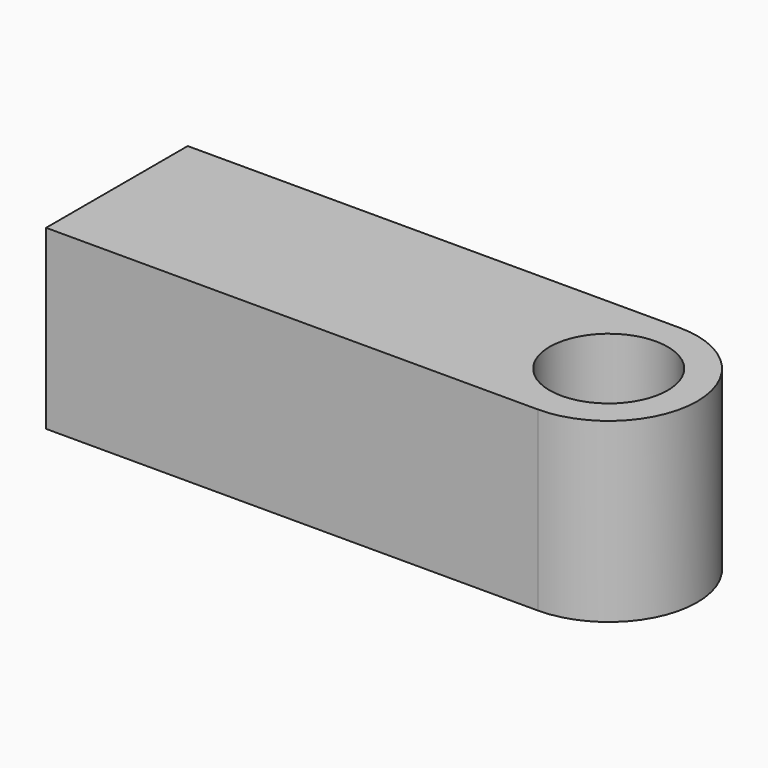
from build123d import *

# Parameters (mm, degrees)
F1_DEPTH = 9
F2_W     = 6
F2_H     = 6
F3_DEPTH = 10


# Not quite as in the source:
# - a feature names something its author has since deleted; it is built from what else it names


with BuildPart() as f1:
    # F0 (on Top) → F1 (new body)
    with BuildSketch(Plane.XY):
        with BuildLine():
            Line((-25, -4.5), (0, -4.5))
            ThreePointArc((0, -4.5), (4.5, 0), (0, 4.5))
            Line((0, 4.5), (-25, 4.5))
            Line((-25, 4.5), (-25, 0))
            Line((-25, 0), (-25, -4.5))
        make_face()
        with BuildLine():
            ThreePointArc((3, 0), (0, -3), (-3, 0))
            ThreePointArc((-3, 0), (0, 3), (3, 0))
        make_face(mode=Mode.SUBTRACT)
    extrude(amount=F1_DEPTH)

    # F2 (on face) → F3 (cut)
    with BuildSketch(Plane(origin=(-25, 0, 0), x_dir=(0, -1, 0), z_dir=(-1, 0, 0))):
        with Locations((0, 4.5)):
            Rectangle(F2_W, F2_H)
    extrude(amount=-F3_DEPTH, mode=Mode.SUBTRACT)


solid = f1.part
